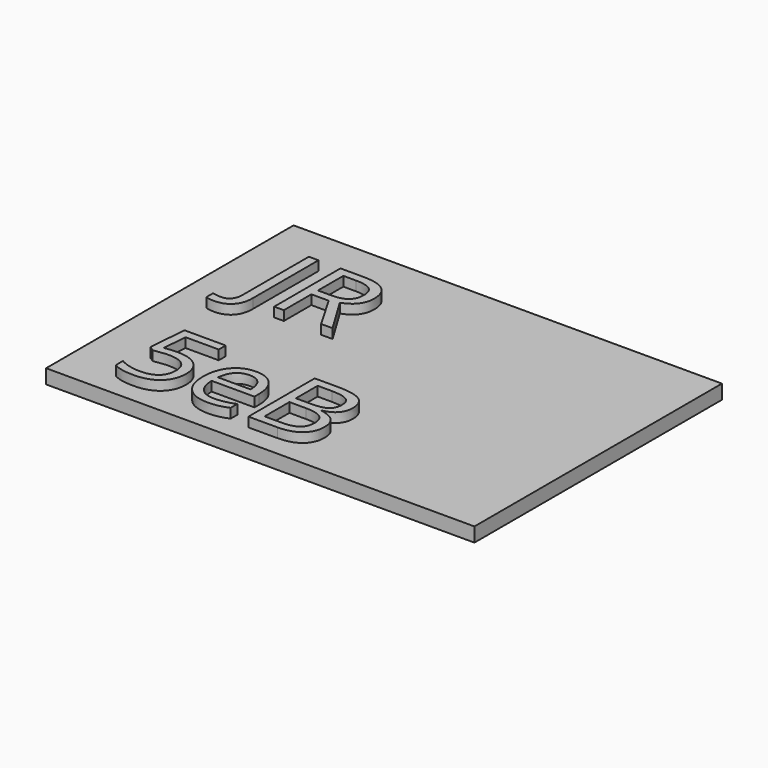
from build123d import *

# Parameters (mm, degrees)
F0_W         = 90
F0_H         = 65
F1_DEPTH     = 3
F2_TEXT_SIZE = 24.3788209951
F3_DEPTH     = 2


# Not quite as in the source:
# - Text() gives the source's letters only with a copy of the font that has no kerning and outlines rounded to 1/6400 em; it was checked with that copy


with BuildPart() as f1:
    # F0 (on Top) → F1 (new body)
    with BuildSketch(Plane.XY):
        with Locations((45, -32.5)):
            Rectangle(F0_W, F0_H)
    extrude(amount=F1_DEPTH)

    # F2 (on face) → F3 (join)
    with BuildSketch(Plane.XY.offset(3)):
        with Locations((9.057928808, -27.5408364832)):
            Text('JR', F2_TEXT_SIZE, font='Open Sans', text_align=(TextAlign.LEFT, TextAlign.BOTTOM))
        with Locations((9.057928808, -60.6960330365)):
            Text('5eB', F2_TEXT_SIZE, font='Open Sans', text_align=(TextAlign.LEFT, TextAlign.BOTTOM))
    extrude(amount=F3_DEPTH)


solid = f1.part
